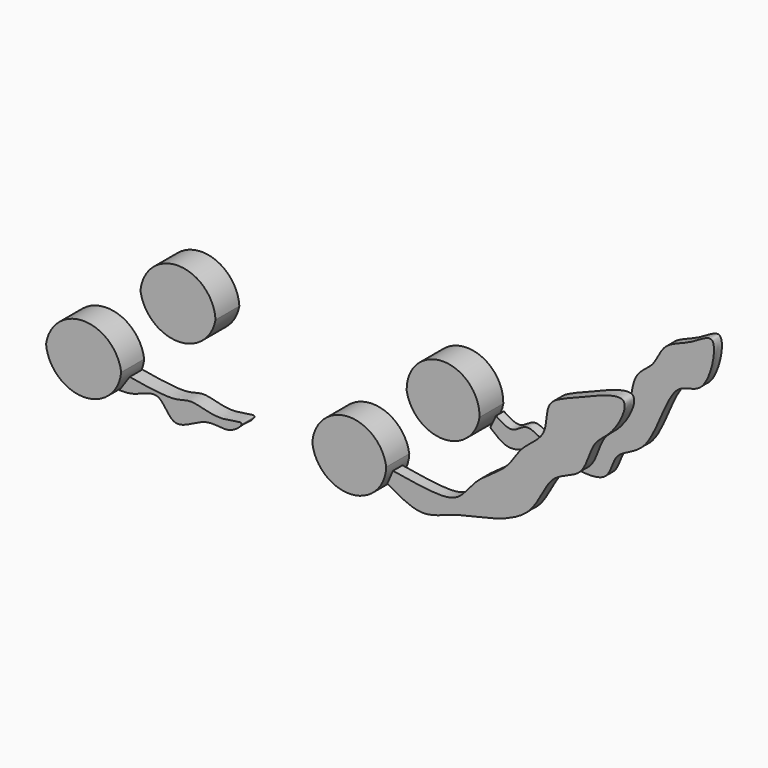
from build123d import *

# Parameters (mm, degrees)
F3_DEPTH  = 7.62
F5_START  = 30.48
F5_DEPTH  = 7.366
F10_START = 32.512
F10_DEPTH = 4.064
F12_DEPTH = 2.54
F14_START = 32.766
F14_DEPTH = 3.048


# Not quite as in the source:
# - a feature of the source that left no trace in its solid (it failed there, or was rolled back) is left out


with BuildPart() as f3:
    # F2 (on Front) → F3 (new body)
    with BuildSketch(Plane.XZ):
        with BuildLine():
            ThreePointArc((-32.0622958243, -31.042130664), (-22.5671676861, -39.3428580499), (-12.8249181435, -31.3336066902))
            ThreePointArc((-12.8249181435, -31.3336066902), (-22.3079495267, -22.2344951449), (-32.0622958243, -31.042130664))
        make_face()
    extrude(amount=F3_DEPTH)


with BuildPart() as f3b:
    # F2 (on Front) → F3, piece 2 (new body)
    with BuildSketch(Plane.XZ):
        with BuildLine():
            ThreePointArc((54.7973737121, -31.3336066902), (45.4701632261, -21.7478670021), (36.1429527402, -31.3336066902))
            ThreePointArc((36.1429527402, -31.3336066902), (45.4701632261, -39.2552673611), (54.7973737121, -31.3336066902))
        make_face()
    extrude(amount=F3_DEPTH)


with BuildPart() as f5:
    # F4 (on Front) → F5 (new body)
    with BuildSketch(Plane.XZ.offset(F5_START)):
        with BuildLine():
            ThreePointArc((55.0888516009, -30.1677044481), (45.3544980302, -21.9635651251), (36.1429527402, -30.7506565005))
            ThreePointArc((36.1429527402, -30.7506565005), (45.8865592043, -39.2555141814), (55.0888516009, -30.1677044481))
        make_face()
    extrude(amount=F5_DEPTH)


with BuildPart() as f5b:
    # F4 (on Front) → F5, piece 2 (new body)
    with BuildSketch(Plane.XZ.offset(F5_START)):
        with BuildLine():
            ThreePointArc((-32.0622958243, -30.7506565005), (-22.50643221, -39.5846133097), (-12.8249181435, -30.8885447899))
            ThreePointArc((-12.8249181435, -30.8885447899), (-22.3834626351, -22.4286085081), (-32.0622958243, -30.7506565005))
        make_face()
    extrude(amount=F5_DEPTH)


with BuildPart() as f10:
    # F9 (on Front) → F10 (new body)
    with BuildSketch(Plane.XZ.offset(F10_START)):
        with BuildLine():
            Line((-11.6430511698, -32.0522002876), (-14.2939854413, -35.9081029892))
            add(Edge.make_bspline(
                [(-14.2939854413, -35.9081029892), (-13.0261920226, -35.9217985745), (-10.2411730767, -35.9518842841), (-3.6972167895, -32.067176477), (-0.6526611469, -41.4878923356), (7.9354953161, -34.2437685404), (13.6886514938, -37.062622216), (19.0468557998, -31.9439594198), (11.0166528887, -34.8102692246), (4.2357707624, -31.7017673976), (-0.1019163298, -34.0328198043), (-7.2173430278, -32.8117134587), (-11.6430511698, -32.0522002876)],
                knots=[0, 0, 0, 0, 0.0817804158, 0.1796507254, 0.2798147687, 0.3958981984, 0.496725844, 0.5748490351, 0.6677536759, 0.7785184426, 0.8622411876, 1, 1, 1, 1], degree=3))
        make_face()
    extrude(amount=F10_DEPTH)


with BuildPart() as f12:
    # F11 (on Front) → F12 (new body)
    with BuildSketch(Plane.XZ):
        with BuildLine():
            Line((54.9466274679, -33.0161750317), (53.5006634891, -36.1490957439))
            add(Edge.make_bspline(
                [(53.5006634891, -36.1490957439), (55.0977031822, -37.5291051807), (58.4971096899, -40.4665481762), (65.95231419, -36.0829829107), (75.220780577, -38.6590857149), (84.2740446829, -38.8614831079), (84.9867128408, -30.5704887045), (95.0561453643, -29.442146953), (99.5642019357, -9.1984577723), (108.9775737416, -12.1162628564), (112.6514347043, 5.4757828233), (104.7356559767, -0.9054966333), (97.610048844, -2.2872474322), (95.5809065439, -9.2212217621), (89.1264094725, -11.5761250504), (89.5907046652, -25.9562030628), (80.7127857094, -20.3681681585), (79.6370960355, -29.4117745628), (71.7883024771, -28.8151287093), (68.8548746122, -37.0011474599), (62.9953508407, -31.3612877239), (59.3615184452, -35.9387020137), (56.4427299675, -34.0065505462), (54.9466274679, -33.0161750317)],
                knots=[0, 0, 0, 0, 0.0428995105, 0.0913144962, 0.1473010549, 0.1960692943, 0.2397362956, 0.2915096473, 0.3655619931, 0.4122404563, 0.472230596, 0.514435054, 0.5632406868, 0.6070632899, 0.6516890708, 0.7088970126, 0.7507505853, 0.7945731891, 0.840160914, 0.8841715253, 0.9252120043, 0.9616654279, 1, 1, 1, 1], degree=3))
        make_face()
    extrude(amount=F12_DEPTH)


with BuildPart() as f14:
    # F13 (on Front) → F14 (new body)
    with BuildSketch(Plane.XZ.offset(F14_START)):
        with BuildLine():
            Line((55.1867857575, -31.8112075329), (53.7408217788, -35.1851209998))
            add(Edge.make_bspline(
                [(53.7408217788, -35.1851209998), (56.7689637452, -36.9330334514), (62.5087672191, -40.2461786318), (70.2592065444, -36.4157693672), (78.7726962572, -34.9327520704), (91.613253656, -31.0834116118), (94.9125403625, -18.8195115021), (104.3924592621, -17.8839546306), (105.9953471436, -8.1326839767), (111.4982887953, -5.8845986156), (117.8826794999, 6.9760166295), (101.6285454747, -0.5279137667), (93.9136567912, -2.8374317125), (95.1194571248, -11.4614076745), (87.702528516, -15.4749706319), (84.8232437703, -22.0961772874), (76.0186806364, -26.5229741761), (72.1474950288, -33.9102753728), (62.8915004783, -33.097073848), (57.7463494376, -32.2383819107), (55.1867857575, -31.8112075329)],
                knots=[0, 0, 0, 0, 0.0589219677, 0.1116858188, 0.1684910819, 0.2356671119, 0.2989431452, 0.3518989619, 0.405905123, 0.4542432276, 0.508758212, 0.5757840676, 0.6298501395, 0.6788924148, 0.7309068655, 0.7813024638, 0.8396904696, 0.8917049158, 0.946126331, 1, 1, 1, 1], degree=3))
        make_face()
    extrude(amount=F14_DEPTH)


solid = Compound([f3.part, f3b.part, f5.part, f5b.part, f10.part, f12.part, f14.part])
